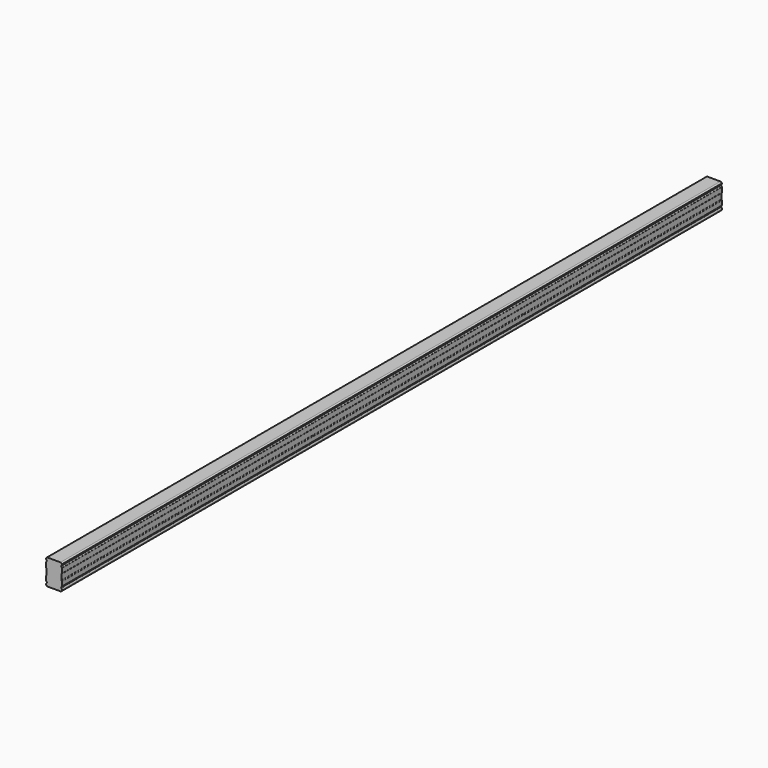
from build123d import *

# Parameters (mm, degrees)
F1_DEPTH = 1364


# Not quite as in the source:
# - a feature of the source that left no trace in its solid (it failed there, or was rolled back) is left out
# - a pattern or mirror of a feature is missing from the dataset's text; its kind, count and spacing are read off the source's solid


with BuildPart() as f1:
    # F0 (on Front) → F1 (new body)
    with BuildSketch(Plane.XZ):
        with BuildLine():
            Line((-26.1803913116, 65.7064561546), (-66.3712014047, 65.7064561546))
            ThreePointArc((-66.3712014047, 65.7064561546), (-69.3844645404, 64.6964743594), (-71.1803913116, 62.0745542645))
            ThreePointArc((-71.1803913116, 62.0745542645), (-70.7044517023, 59.6823321584), (-69.349118798, 57.6544470937))
            ThreePointArc((-69.349118798, 57.6544470937), (-68.8489055801, 56.8195085607), (-68.802041246, 55.8473257839))
            ThreePointArc((-68.802041246, 55.8473257839), (-69.4413893704, 54.0856160437), (-70.5743109736, 52.592674024))
            ThreePointArc((-70.5743109736, 52.592674024), (-71.0226507022, 51.9369653038), (-71.1803913116, 51.1584536867))
            Line((-71.1803913116, 51.1584536867), (-71.1803913116, 37.1704536867))
            ThreePointArc((-71.1803913116, 37.1704536867), (-70.9124421192, 36.1704536867), (-70.1803913116, 35.4384028791))
            ThreePointArc((-70.1803913116, 35.4384028791), (-69.4483405041, 34.7063520715), (-69.1803913116, 33.7063520715))
            Line((-69.1803913116, 33.7063520715), (-69.1803913116, 17.7064561546))
            ThreePointArc((-69.1803913116, 17.7064561546), (-69.4483405041, 16.7064561546), (-70.1803913116, 15.974405347))
            ThreePointArc((-70.1803913116, 15.974405347), (-70.9124421192, 15.2423545394), (-71.1803913116, 14.2423545394))
            Line((-71.1803913116, 14.2423545394), (-71.1803913116, 1.6428347462))
            ThreePointArc((-71.1803913116, 1.6428347462), (-71.017419076, 0.8520572851), (-70.5550623187, 0.1901545948))
            ThreePointArc((-70.5550623187, 0.1901545948), (-69.4072427397, -1.3029633413), (-68.7788291433, -3.0783470488))
            ThreePointArc((-68.7788291433, -3.0783470488), (-68.8366723002, -4.0382506294), (-69.3358356782, -4.8601974871))
            ThreePointArc((-69.3358356782, -4.8601974871), (-70.7008560802, -6.8926614338), (-71.1803913116, -9.2935438454))
            ThreePointArc((-71.1803913116, -9.2935438454), (-69.7159252176, -12.8290777513), (-66.1803913116, -14.2935438454))
            Line((-66.1803913116, -14.2935438454), (-26.3712014047, -14.2935438454))
            ThreePointArc((-26.3712014047, -14.2935438454), (-22.8356674987, -12.8290777513), (-21.3712014047, -9.2935438454))
            ThreePointArc((-21.3712014047, -9.2935438454), (-21.8507366361, -6.8926614338), (-23.2157570381, -4.8601974871))
            ThreePointArc((-23.2157570381, -4.8601974871), (-23.7149204161, -4.0382506294), (-23.772763573, -3.0783470488))
            ThreePointArc((-23.772763573, -3.0783470488), (-23.1443499766, -1.3029633413), (-21.9965303976, 0.1901545948))
            ThreePointArc((-21.9965303976, 0.1901545948), (-21.5341736403, 0.8520572851), (-21.3712014047, 1.6428347462))
            Line((-21.3712014047, 1.6428347462), (-21.3712014047, 14.2423545394))
            ThreePointArc((-21.3712014047, 14.2423545394), (-21.6391505971, 15.2423545394), (-22.3712014047, 15.974405347))
            ThreePointArc((-22.3712014047, 15.974405347), (-23.1032522122, 16.7064561546), (-23.3712014047, 17.7064561546))
            Line((-23.3712014047, 17.7064561546), (-23.3712014047, 33.7063520715))
            ThreePointArc((-23.3712014047, 33.7063520715), (-23.1032522122, 34.7063520715), (-22.3712014047, 35.4384028791))
            ThreePointArc((-22.3712014047, 35.4384028791), (-21.6391505971, 36.1704536867), (-21.3712014047, 37.1704536867))
            Line((-21.3712014047, 37.1704536867), (-21.3712014047, 51.1584536867))
            ThreePointArc((-21.3712014047, 51.1584536867), (-21.5289420141, 51.9369653038), (-21.9772817427, 52.592674024))
            ThreePointArc((-21.9772817427, 52.592674024), (-23.1102033459, 54.0856160437), (-23.7495514703, 55.8473257839))
            ThreePointArc((-23.7495514703, 55.8473257839), (-23.7026871362, 56.8195085607), (-23.2024739183, 57.6544470937))
            ThreePointArc((-23.2024739183, 57.6544470937), (-21.847141014, 59.6823321584), (-21.3712014047, 62.0745542645))
            ThreePointArc((-21.3712014047, 62.0745542645), (-23.1671281759, 64.6964743594), (-26.1803913116, 65.7064561546))
        make_face()
    extrude(amount=F1_DEPTH)

    # F1_copies: F1 across plane


with BuildPart() as f1_1:
    add(f1.part)
    add(f1.part.mirror(Plane(origin=(0, -1291.5, 0), x_dir=(0, 0, -1), z_dir=(0, -1, 0))))


solid = f1_1.part
